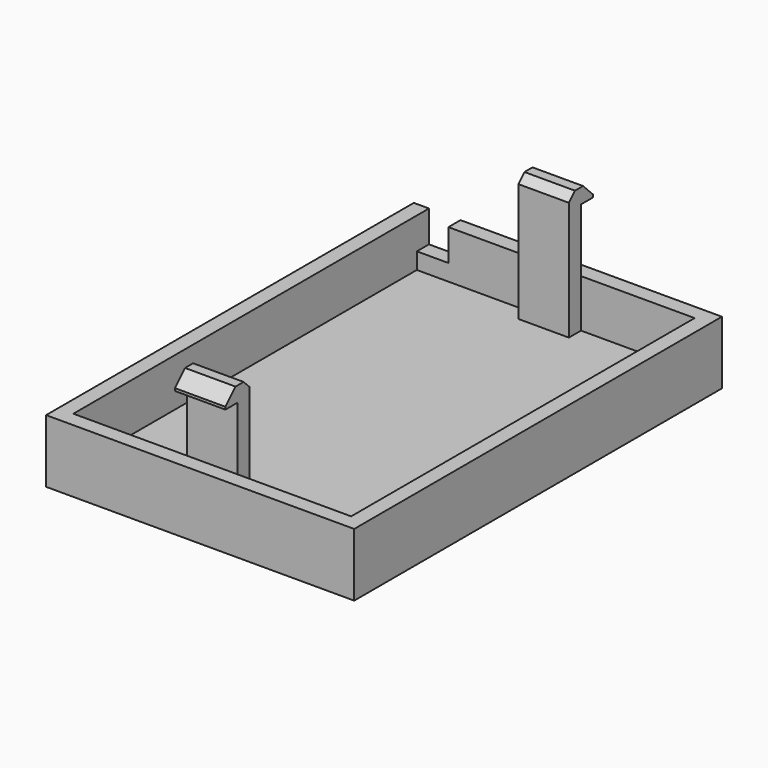
from build123d import *

# Parameters (mm, degrees)
F0_W      = 22
F0_H      = 34
F1_DEPTH  = 1.2
F0_W_2    = 24.4
F0_H_2    = 36.4
F2_DEPTH  = 5
F3_W      = 4
F3_H      = 6.2
F3_H_2    = 3.8
F4_DEPTH  = 1.2
F5_SIZE   = 0.6
F6_W      = 4
F6_H      = 1.2
F7_DEPTH  = 1.2
F8_SIZE   = 1
F9_W      = 2.5
F9_H      = 2.5
F10_DEPTH = 25


# Not quite as in the source:
# - a pattern or mirror of a feature is missing from the dataset's text; its kind, count and spacing are read off the source's solid


with BuildPart() as f1:
    # F0 (on Top) → F1 (new body)
    with BuildSketch(Plane.XY):
        Rectangle(F0_W, F0_H)
    extrude(amount=F1_DEPTH)

    # F0 (on Top) → F2 (join)
    with BuildSketch(Plane.XY):
        Rectangle(F0_W_2, F0_H_2)
        Rectangle(F0_W, F0_H, mode=Mode.SUBTRACT)
    extrude(amount=F2_DEPTH)

    # F3 (on face) → F4 (join)
    with BuildSketch(Plane(origin=(0, -17, 0), x_dir=(-1, 0, 0), z_dir=(0, 1, 0))):
        with Locations((0, 8.1)):
            Rectangle(F3_W, F3_H)
        with Locations((0, 3.1)):
            Rectangle(F3_W, F3_H_2)
    f4 = extrude(amount=F4_DEPTH)

    # F4_copies: F4 across plane
    add(f4.mirror(Plane.ZX))

    # F5
    f5_edges = [f1.edges().sort_by_distance(p)[0] for p in [
        (0, -15.8, 11.2),
        (0, 15.8, 11.2),
    ]]
    chamfer(f5_edges, length=F5_SIZE)

    # F6 (on face) → F7 (join)
    with BuildSketch(Plane.XZ.offset(17)):
        with Locations((0, 10.6)):
            Rectangle(F6_W, F6_H)
    f7 = extrude(amount=F7_DEPTH)

    # F7_copies: F7 across plane
    add(f7.mirror(Plane.ZX))

    # F8
    f8_edges = [f1.edges().sort_by_distance(p)[0] for p in [
        (0, -18.2, 11.2),
        (0, 18.2, 11.2),
    ]]
    chamfer(f8_edges, length=F8_SIZE)

    # F9 (on face) → F10 (cut)
    with BuildSketch(Plane.XZ.offset(-17)):
        with Locations((-9.75, 3.75)):
            Rectangle(F9_W, F9_H)
    extrude(amount=-F10_DEPTH, mode=Mode.SUBTRACT)


solid = f1.part
